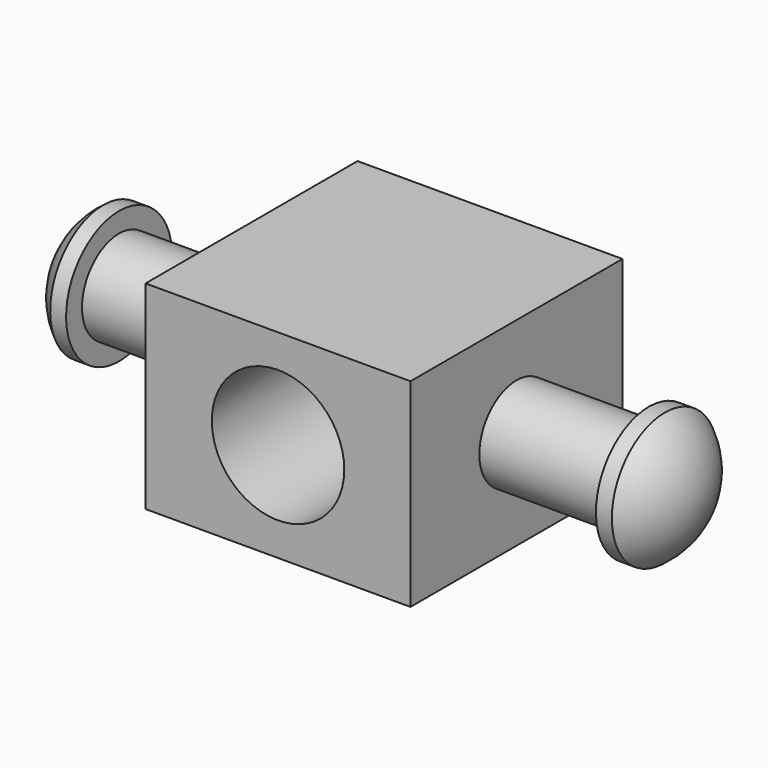
from build123d import *

# Parameters (mm, degrees)
F1_DEPTH = 5
F0_W     = 5
F0_H     = 1.75
F5_R     = 2.5
F6_DEPTH = 25


# Not quite as in the source:
# - a pattern or mirror of a feature is missing from the dataset's text; its kind, count and spacing are read off the source's solid
# - a feature names something its author has since deleted; it is built from what else it names


with BuildPart() as f1:
    # F0 (on Front) → F1 (new body, symmetric)
    with BuildSketch(Plane.XZ):
        Polygon((5, 1.75), (5, 3.75), (-5, 3.75), (-5, -3.75), (5, -3.75), (5, 0), align=None)
    extrude(amount=F1_DEPTH, both=True)

    # F0 (on Front) → F2 (revolve)
    with BuildSketch(Plane.XZ):
        with Locations((7.5, 0.875)):
            Rectangle(F0_W, F0_H)
    f2 = revolve(axis=Axis((7.5, 0, 0), (1, 0, 0)))

    # F2_copies: F2 across plane
    add(f2.mirror(Plane(origin=(0, 0, 0), x_dir=(0, 0, -1), z_dir=(-1, 0, 0))))

    # F0 (on Front) → F3 (revolve)
    with BuildSketch(Plane.XZ):
        Polygon((10, 2.5), (10, 1.75), (10, 0), (10.6, 0), (10.6, 2.5), align=None)
    f3 = revolve(axis=Axis((12.1656447835, 0, 0), (1, 0, 0)))

    # F3_copies: F3 across plane
    add(f3.mirror(Plane(origin=(0, 0, 0), x_dir=(0, 0, -1), z_dir=(-1, 0, 0))))

    # F0 (on Front) → F4 (revolve)
    with BuildSketch(Plane.XZ):
        with BuildLine():
            Line((10.6, 2.5), (10.6, 0))
            Line((10.6, 0), (11.9, 0))
            ThreePointArc((11.9, 0), (11.5555774622, 1.4089002804), (10.6, 2.5))
        make_face()
    f4 = revolve(axis=Axis((12.1656447835, 0, 0), (1, 0, 0)))

    # F4_copies: F4 across plane
    add(f4.mirror(Plane(origin=(0, 0, 0), x_dir=(0, 0, -1), z_dir=(-1, 0, 0))))

    # F5 (on face) → F6 (cut)
    with BuildSketch(Plane.XZ.offset(5)):
        Circle(F5_R)
    extrude(amount=-F6_DEPTH, mode=Mode.SUBTRACT)


solid = f1.part
